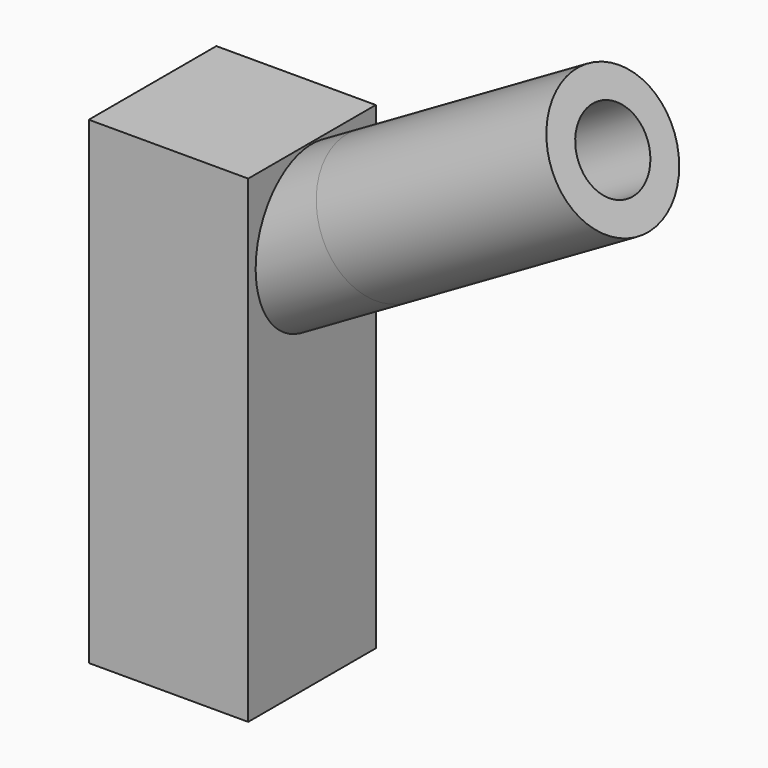
from build123d import *

# Parameters (mm, degrees)
F0_W      = 6
F0_H      = 6
F0_R      = 2.05
F1_DEPTH  = 15
F3_W      = 6
F3_H      = 6
F4_DEPTH  = 3
F8_R      = 2.65
F8_R_2    = 1.5
F10_DEPTH = 10
F11_DEPTH = 8.02


with BuildPart() as f1:
    # F0 (on Top) → F1 (new body)
    with BuildSketch(Plane.XY):
        Rectangle(F0_W, F0_H)
        Circle(F0_R, mode=Mode.SUBTRACT)
    extrude(amount=F1_DEPTH)

    # F3 (on offset) → F4 (join)
    with BuildSketch(Plane.XY.offset(15)):
        Rectangle(F3_W, F3_H)
    extrude(amount=F4_DEPTH)

    # F8 (on offset) → F9 (join, up to the next surface of F1)
    with BuildSketch(Plane(origin=(11.349514303, 0, 6.552645138), x_dir=(0, -1, 0), z_dir=(-0.8660254038, 0, -0.5))):
        with Locations((0, 11.3801583648)):
            Circle(F8_R)
        with Locations((0, 11.3801583648)):
            Circle(F8_R_2, mode=Mode.SUBTRACT)
    extrude(until=Until.NEXT)

    # F8 (on offset) → F10 (join)
    with BuildSketch(Plane(origin=(11.349514303, 0, 6.552645138), x_dir=(0, -1, 0), z_dir=(-0.8660254038, 0, -0.5))):
        with Locations((0, 11.3801583648)):
            Circle(F8_R)
        with Locations((0, 11.3801583648)):
            Circle(F8_R_2, mode=Mode.SUBTRACT)
    extrude(amount=-F10_DEPTH)

    # F8 (on offset) → F11 (cut)
    with BuildSketch(Plane(origin=(11.349514303, 0, 6.552645138), x_dir=(0, -1, 0), z_dir=(-0.8660254038, 0, -0.5))):
        with Locations((0, 11.3801583648)):
            Circle(F8_R_2)
    extrude(amount=F11_DEPTH, mode=Mode.SUBTRACT)


solid = f1.part
